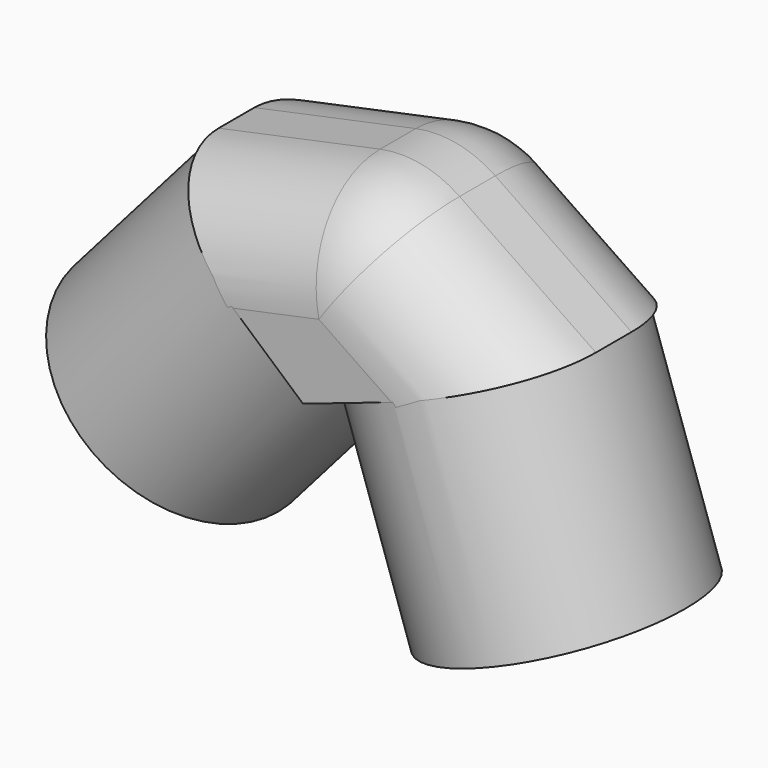
from build123d import *

# Parameters (mm, degrees)
F2_R          = 14.2875
F2_R_2        = 11.43
F5_R          = 14.2875
F5_R_2        = 11.43
F7_DEPTH      = 14.2875
F7_DEPTH_BACK = 14.2875
F8_T1_DEPTH   = 48.1632201407
F8_T3_DEPTH   = 48.1632201407
F8_T5_DEPTH   = 5.08
F8_T10_DEPTH  = 11.7475
F8_T16_DEPTH  = 11.7475


# Not quite as in the source:
# - a fillet or chamfer that OpenCascade refuses, or shapes differently, is made with other operations: its cross-section is extruded or revolved along the edge and cut away or added


with BuildPart() as f3:
    # F3: sweep along a path in F0
    with BuildLine(Plane.XZ) as f3_path:
        Line((43.6000298417, -8.651005595), (35.4240159518, 15.3971294028))
    # F2 (on line) → F3 (sweep)
    with BuildSketch(Plane(origin=(7.1540121537, 0, -21.0421181231), x_dir=(0.9467769684, 0, 0.3218903106), z_dir=(-0.3218903106, 0, 0.9467769684))):
        with Locations((38.471757228, 0)):
            Circle(F2_R)
        with Locations((38.471757228, 0)):
            Circle(F2_R_2, mode=Mode.SUBTRACT)
    sweep(path=f3_path.line)

    # F6: sweep along a path in F0
    with BuildLine(Plane.XZ) as f6_path:
        Line((0, 0), (16.7382888768, 19.1047032292))
    # F5 (on face) → F6 (sweep)
    with BuildSketch(Plane(origin=(0, 0, 0), x_dir=(0.7521536704, 0, -0.6589877511), z_dir=(0.6589877511, 0, 0.7521536704))):
        Circle(F5_R)
        Circle(F5_R_2, mode=Mode.SUBTRACT)
    sweep(path=f6_path.line)

    # F0 (on Front) → F7 (join, two sides)
    with BuildSketch(Plane.XZ) as f7_sk:
        with BuildLine():
            Line((14.1742345569, 21.3511595802), (16.7382888768, 19.1047032292))
            Line((16.7382888768, 19.1047032292), (29.2920055344, 33.4332306512))
            Line((29.2920055344, 33.4332306512), (25.1637988833, 32.5627254125))
            add(Edge.make_bspline(
                [(14.1742345569, 21.3511595802), (18.1555587274, 26.691715757), (21.8910272526, 30.7931889907), (25.1637988833, 32.5627254125)],
                knots=[0.2192972469, 0.2192972469, 0.2192972469, 0.2192972469, 0.4127143591, 0.4127143591, 0.4127143591, 0.4127143591], degree=3))
        make_face()
        Polygon((29.2920055344, 33.4332306512), (16.7382888768, 19.1047032292), (25.0025134025, 11.8539710829), (25.0108680409, 11.8568115377), align=None)
        with BuildLine():
            Line((5.9918933103, 28.5199907224), (14.1742345569, 21.3511595802))
            add(Edge.make_bspline(
                [(14.1742345569, 21.3511595802), (18.1555587274, 26.691715757), (21.8910272526, 30.7931889907), (25.1637988833, 32.5627254125)],
                knots=[0.2192972469, 0.2192972469, 0.2192972469, 0.2192972469, 0.4127143591, 0.4127143591, 0.4127143591, 0.4127143591], degree=3))
            Line((25.1637988833, 32.5627254125), (5.9918933103, 28.5199907224))
        make_face()
        with BuildLine():
            Line((32.7751119786, 31.0525082771), (29.2920055344, 33.4332306512))
            Line((29.2920055344, 33.4332306512), (35.4240159518, 15.3971294028))
            Line((35.4240159518, 15.3971294028), (38.6515313802, 16.4944374051))
            add(Edge.make_bspline(
                [(32.7751119786, 31.0525082771), (35.1243349239, 28.1674701754), (37.0108609747, 22.9504952618), (38.6515313802, 16.4944374051)],
                knots=[0.5872856409, 0.5872856409, 0.5872856409, 0.5872856409, 0.7807027531, 0.7807027531, 0.7807027531, 0.7807027531], degree=3))
        make_face()
        Polygon((35.4240159518, 15.3971294028), (29.2920055344, 33.4332306512), (25.0108680409, 11.8568115377), align=None)
        with BuildLine():
            Line((48.951091888, 19.9961372159), (32.7751119786, 31.0525082771))
            add(Edge.make_bspline(
                [(32.7751119786, 31.0525082771), (35.1243349239, 28.1674701754), (37.0108609747, 22.9504952618), (38.6515313802, 16.4944374051)],
                knots=[0.5872856409, 0.5872856409, 0.5872856409, 0.5872856409, 0.7807027531, 0.7807027531, 0.7807027531, 0.7807027531], degree=3))
            Line((38.6515313802, 16.4944374051), (48.951091888, 19.9961372159))
        make_face()
    extrude(amount=F7_DEPTH)
    extrude(f7_sk.sketch, amount=-F7_DEPTH_BACK)

    # F8: fillet of radius 11.7475 on 5 edges, made by hand

    # F8_s2 → F8_t1 (cut)
    with BuildSketch(Plane(origin=(48.2948087603, 0, -33.0097668872), x_dir=(0, 1, 0), z_dir=(-0.8255784296, 0, 0.5642873884))):
        with BuildLine():
            ThreePointArc((14.2875, -32.3833633586), (10.846736912, -40.6901002706), (2.54, -44.1308633586))
            Line((2.54, -44.1308633586), (14.2875, -44.1308633586))
            Line((14.2875, -44.1308633586), (14.2875, -32.3833633586))
        make_face()
        with BuildLine():
            ThreePointArc((-2.54, -44.1308633586), (-10.846736912, -40.6901002706), (-14.2875, -32.3833633586))
            Line((-14.2875, -32.3833633586), (-14.2875, -44.1308633586))
            Line((-14.2875, -44.1308633586), (-2.54, -44.1308633586))
        make_face()
    extrude(amount=F8_T1_DEPTH, mode=Mode.SUBTRACT)

    # F8_s4 → F8_t3 (cut)
    with BuildSketch(Plane(origin=(29.884780339, 0, 6.3017334256), x_dir=(0, 1, 0), z_dir=(-0.9784824031, 0, -0.2063302857))):
        with BuildLine():
            ThreePointArc((14.2875, -14.9225), (10.846736912, -23.229236912), (2.54, -26.67))
            Line((2.54, -26.67), (14.2875, -26.67))
            Line((14.2875, -26.67), (14.2875, -14.9225))
        make_face()
        with BuildLine():
            ThreePointArc((-14.2875, -14.9225), (-10.846736912, -23.229236912), (-2.54, -26.67))
            Line((-2.54, -26.67), (-14.2875, -26.67))
            Line((-14.2875, -26.67), (-14.2875, -14.9225))
        make_face()
    extrude(amount=F8_T3_DEPTH, mode=Mode.SUBTRACT)

    # F8_s6 → F8_t5 (cut)
    with BuildSketch(Plane.XZ.offset(-2.54)):
        with BuildLine():
            ThreePointArc((33.434782745, 30.6016196872), (29.0921538432, 32.4260021156), (24.3819516188, 32.3978591166))
            Line((24.3819516188, 32.3978591166), (29.2920055344, 33.4332306512))
            Line((29.2920055344, 33.4332306512), (33.434782745, 30.6016196872))
        make_face()
    extrude(amount=F8_T5_DEPTH, mode=Mode.SUBTRACT)


with BuildPart() as f8_tool8:
    # F8_s9 → F8_t10 (new body)
    with BuildSketch(Plane.XZ.offset(-2.54)):
        Polygon((26.8058166503, 20.903137086), (33.434782745, 30.6016196872), (29.2920055344, 33.4332306512), (24.3819516188, 32.3978591166), align=None)
    extrude(amount=-F8_T10_DEPTH)

    # F8_s11 → F8_t12 (revolve, cut)
    with BuildSketch(Plane(origin=(26.8058166503, 2.54, 20.903137086), x_dir=(-0.194623298, 0, -0.9808780617), z_dir=(0.9808780617, 0, -0.194623298))):
        with BuildLine():
            ThreePointArc((0, -11.7475), (11.7475, 0), (0, 11.7475))
            Line((0, 11.7475), (0, -11.7475))
        make_face()
    revolve(axis=Axis((26.8058166503, 2.54, 20.903137086), (0, 1, 0)), mode=Mode.SUBTRACT)


with BuildPart() as f3_1:
    add(f3.part)

    # F8_t7: cut F8_tool8
    add(f8_tool8.part, mode=Mode.SUBTRACT)


with BuildPart() as f8_tool14:
    # F8_s15 → F8_t16 (new body)
    with BuildSketch(Plane.XZ.offset(2.54)):
        Polygon((26.8058166503, 20.903137086), (24.3819516188, 32.3978591166), (29.2920055344, 33.4332306512), (33.434782745, 30.6016196872), align=None)
    extrude(amount=F8_T16_DEPTH)

    # F8_s17 → F8_t18 (revolve, cut)
    with BuildSketch(Plane(origin=(26.8058166503, -2.54, 20.903137086), x_dir=(-0.194623298, 0, -0.9808780617), z_dir=(-0.9808780617, 0, 0.194623298))):
        with BuildLine():
            ThreePointArc((0, -11.7475), (11.7475, 0), (0, 11.7475))
            Line((0, 11.7475), (0, -11.7475))
        make_face()
    revolve(axis=Axis((26.8058166503, -2.54, 20.903137086), (0, -1, 0)), mode=Mode.SUBTRACT)


with BuildPart() as f3_2:
    add(f3_1.part)

    # F8_t13: cut F8_tool14
    add(f8_tool14.part, mode=Mode.SUBTRACT)


solid = f3_2.part
